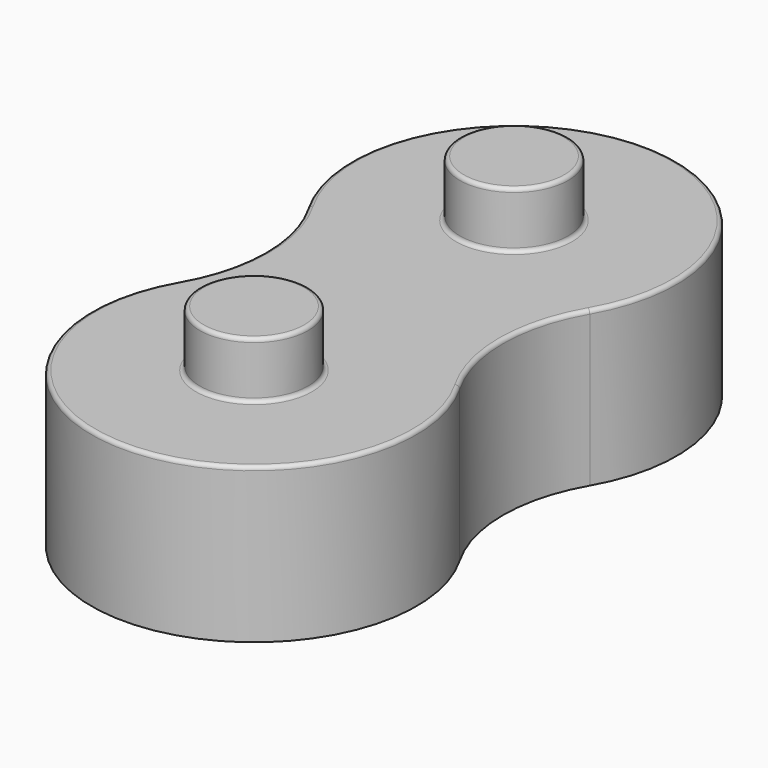
from build123d import *

# Parameters (mm, degrees)
F4_R     = 7.9
F5_DEPTH = 20
F6_DEPTH = 10
F7_R     = 7
F8_DEPTH = 7.3
F9_R     = 0.5


# Not quite as in the source:
# - a feature names something its author has since deleted; it is built from what else it names


with BuildPart() as f5:
    # F4 (on Top) → F5 (new body)
    with BuildSketch(Plane.XY):
        with BuildLine():
            ThreePointArc((18.1865334795, 10.5), (15.3730669589, 21), (18.1865334795, 31.5))
            ThreePointArc((18.1865334795, 31.5), (0, 63), (-18.1865334795, 31.5))
            ThreePointArc((-18.1865334795, 31.5), (-15.3730669589, 21), (-18.1865334795, 10.5))
            ThreePointArc((-18.1865334795, 10.5), (0, -21), (18.1865334795, 10.5))
        make_face()
        Circle(F4_R, mode=Mode.SUBTRACT)
        with Locations((0, 42)):
            Circle(F4_R, mode=Mode.SUBTRACT)
        with Locations((0, 42)):
            Circle(F4_R)
        Circle(F4_R)
    extrude(amount=F5_DEPTH)

    # F4 (on Top) → F6 (cut)
    with BuildSketch(Plane.XY):
        with Locations((0, 42)):
            Circle(F4_R)
        Circle(F4_R)
    extrude(amount=F6_DEPTH, mode=Mode.SUBTRACT)

    # F7 (on face) → F8 (join)
    with BuildSketch(Plane.XY.offset(20)):
        Circle(F7_R)
        with Locations((0, 42)):
            Circle(F7_R)
    extrude(amount=F8_DEPTH)

    # F9
    f9_edges = [f5.edges().sort_by_distance(p)[0] for p in [
        (-7, 0, 27.3),
        (-7.9, 42, 0),
        (-7.9, 42, 10),
        (-7.9, 0, 0),
        (-7.9, 0, 10),
        (-7, 42, 27.3),
        (-7, 42, 20),
        (0, 63, 20),
        (-7, 0, 20),
    ]]
    fillet(f9_edges, radius=F9_R)


solid = f5.part
